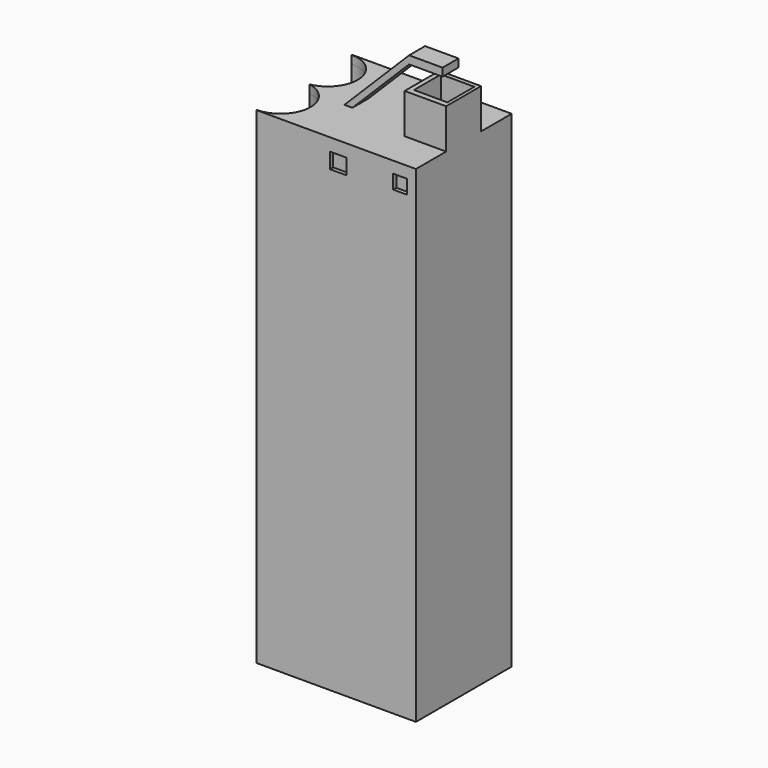
from build123d import *

# Parameters (mm, degrees)
F1_DEPTH  = 76.2
F2_T      = -1.27
F4_DEPTH  = 76.2
F6_DEPTH  = 12.7
F8_DEPTH  = 1.27
F10_DEPTH = 1.27
F12_DEPTH = 1.5875
F13_W     = 6.6033280455
F13_H     = 6.9497893564
F13_W_2   = 5.3267844487
F13_H_2   = 5.3683998995
F14_DEPTH = 6.35
F15_W     = 2.0411710721
F15_H     = 2.829067409
F15_W_2   = 2.1245945245
F15_H_2   = 2.8308555484
F16_DEPTH = 0.635
F17_W     = 2.6483945549
F17_H     = 2.4718344212
F17_W_2   = 2.1775695495
F17_H_2   = 2.236418426
F18_DEPTH = 0.635


# Not quite as in the source:
# - a feature names something its author has since deleted; it is built from what else it names


with BuildPart() as f1:
    # F0 (on Top) → F1 (new body)
    with BuildSketch(Plane.XY):
        with BuildLine():
            Line((0, -9.525), (0, 9.525))
            Line((0, 9.525), (-25.4, 9.525))
            Line((-25.4, 9.525), (-25.4, 9.4535289675))
            ThreePointArc((-25.4, 9.4535289675), (-22.0324039546, 8.0586250129), (-20.6375, 4.6910289675))
            ThreePointArc((-20.6375, 4.6910289675), (-21.7533513451, 1.6278019374), (-24.5780185671, 0))
            ThreePointArc((-24.5780185671, 0), (-21.7533513451, -1.6278019374), (-20.6375, -4.6910289675))
            ThreePointArc((-20.6375, -4.6910289675), (-22.0324039546, -8.0586250129), (-25.4, -9.4535289675))
            Line((-25.4, -9.4535289675), (-25.4, -9.525))
            Line((-25.4, -9.525), (0, -9.525))
        make_face()
    extrude(amount=F1_DEPTH)

    # F2
    f2_openings = [f1.faces().sort_by_distance(p)[0] for p in [
        (-10.85856, 0, 76.2),
    ]]
    offset(amount=F2_T, openings=f2_openings)

    # F3 (on Top) → F4 (join)
    with BuildSketch(Plane.XY):
        with BuildLine():
            Line((-1.27, 1.8135049587), (-1.27, 2.6920572227))
            ThreePointArc((-1.27, 2.6920572227), (-3.9620572227, 0), (-1.27, -2.6920572227))
            Line((-1.27, -2.6920572227), (-1.27, -1.8135049587))
            ThreePointArc((-1.27, -1.8135049587), (-3.0835049587, 0), (-1.27, 1.8135049587))
        make_face()
    extrude(amount=F4_DEPTH)

    # F5 (on face) → F6 (cut)
    with BuildSketch(Plane(origin=(-1.27, 0, 0), x_dir=(0, -1, 0), z_dir=(-1, 0, 0))):
        Polygon((-2.6920572227, 1.27), (2.6920572227, 1.27), (2.6920572227, 10.6323556975), (-3.4403376048, 10.6323556975), (-3.4403376048, 1.27), align=None)
    extrude(amount=F6_DEPTH, mode=Mode.SUBTRACT)

    # F7 (on face) → F8 (join)
    with BuildSketch(Plane.XY.offset(76.2)):
        with BuildLine():
            Line((0, -9.525), (0, 9.525))
            Line((0, 9.525), (-25.4, 9.525))
            Line((-25.4, 9.525), (-25.4, 9.4535289675))
            ThreePointArc((-25.4, 9.4535289675), (-20.6554014022, 5.1035703547), (-24.5780185671, 0))
            ThreePointArc((-24.5780185671, 0), (-20.6554014022, -5.1035703547), (-25.4, -9.4535289675))
            Line((-25.4, -9.4535289675), (-25.4, -9.525))
            Line((-25.4, -9.525), (0, -9.525))
        make_face()
        with BuildLine():
            ThreePointArc((-1.27, 2.6920572227), (-3.9620572227, 0), (-1.27, -2.6920572227))
            Line((-1.27, -2.6920572227), (-1.27, -8.255))
            Line((-1.27, -8.255), (-20.5328481912, -8.255))
            ThreePointArc((-20.5328481912, -8.255), (-19.4179492319, -3.9124887578), (-21.6072037392, 0))
            ThreePointArc((-21.6072037392, 0), (-19.4179492319, 3.9124887578), (-20.5328481912, 8.255))
            Line((-20.5328481912, 8.255), (-1.27, 8.255))
            Line((-1.27, 8.255), (-1.27, 2.6920572227))
        make_face(mode=Mode.SUBTRACT)
        with BuildLine():
            ThreePointArc((-1.27, -1.8135049587), (-3.0835049587, 0), (-1.27, 1.8135049587))
            Line((-1.27, 1.8135049587), (-1.27, -1.8135049587))
        make_face(mode=Mode.SUBTRACT)
        with BuildLine():
            Line((-1.27, -8.255), (-1.27, -2.6920572227))
            ThreePointArc((-1.27, -2.6920572227), (-3.9620572227, 0), (-1.27, 2.6920572227))
            Line((-1.27, 2.6920572227), (-1.27, 8.255))
            Line((-1.27, 8.255), (-20.5328481912, 8.255))
            ThreePointArc((-20.5328481912, 8.255), (-19.4179492319, 3.9124887578), (-21.6072037392, 0))
            ThreePointArc((-21.6072037392, 0), (-19.4179492319, -3.9124887578), (-20.5328481912, -8.255))
            Line((-20.5328481912, -8.255), (-1.27, -8.255))
        make_face()
    extrude(amount=F8_DEPTH)

    # F9 (on face) → F10 (cut)
    with BuildSketch(Plane.XY.offset(77.47)):
        with BuildLine():
            ThreePointArc((-1.8017621012, -1.7337904437), (-3.0835049587, 0), (-1.8017621012, 1.7337904437))
            ThreePointArc((-1.8017621012, 1.7337904437), (-5.239634374, 0), (-1.8017621012, -1.7337904437))
        make_face()
        with BuildLine():
            ThreePointArc((-1.27, -1.1662306034), (-1.0148042261, -0.6077592736), (-0.9273755434, 0))
            ThreePointArc((-0.9273755434, 0), (-1.0148042261, 0.6077592736), (-1.27, 1.1662306034))
            Line((-1.27, 1.1662306034), (-1.27, -1.1662306034))
        make_face()
        with BuildLine():
            Line((-1.27, -1.1662306034), (-1.27, 1.1662306034))
            ThreePointArc((-1.27, 1.1662306034), (-1.5100785054, 1.4741856232), (-1.8017621012, 1.7337904437))
            ThreePointArc((-1.8017621012, 1.7337904437), (-3.0835049587, 0), (-1.8017621012, -1.7337904437))
            ThreePointArc((-1.8017621012, -1.7337904437), (-1.5100785054, -1.4741856232), (-1.27, -1.1662306034))
        make_face()
    extrude(amount=-F10_DEPTH, mode=Mode.SUBTRACT)

    # F11 (on Front) → F12 (join, symmetric)
    with BuildSketch(Plane.XZ):
        Polygon((-7.4378219433, 87.7572894096), (-17.725111353, 77.47), (-16.455111353, 77.47), (-7.4378219433, 86.4872894096), (-2.1149073727, 86.4872894096), (-2.1149073727, 87.7572894096), align=None)
    extrude(amount=F12_DEPTH, both=True)

    # F13 (on face) → F14 (join)
    with BuildSketch(Plane.XY.offset(77.47)):
        with Locations((-3.3016640227, -0.0416187104)):
            Rectangle(F13_W, F13_H)
        with Locations((-3.1908567762, 0.0832278747)):
            Rectangle(F13_W_2, F13_H_2, mode=Mode.SUBTRACT)
    extrude(amount=F14_DEPTH)

    # F15 (on face) → F16 (cut)
    with BuildSketch(Plane(origin=(0, 9.525, 0), x_dir=(-1, 0, 0), z_dir=(0, 1, 0))):
        with Locations((2.4719407083, 74.3873603642)):
            Rectangle(F15_W, F15_H)
        with Locations((11.8596078828, 73.9940367639)):
            Rectangle(F15_W_2, F15_H_2)
    extrude(amount=-F16_DEPTH, mode=Mode.SUBTRACT)

    # F17 (on face) → F18 (cut)
    with BuildSketch(Plane.XZ.offset(9.525)):
        with Locations((-12.3509913683, 74.2306262255)):
            Rectangle(F17_W, F17_H)
        with Locations((-2.5225046556, 74.5248906314)):
            Rectangle(F17_W_2, F17_H_2)
    extrude(amount=-F18_DEPTH, mode=Mode.SUBTRACT)


solid = f1.part
